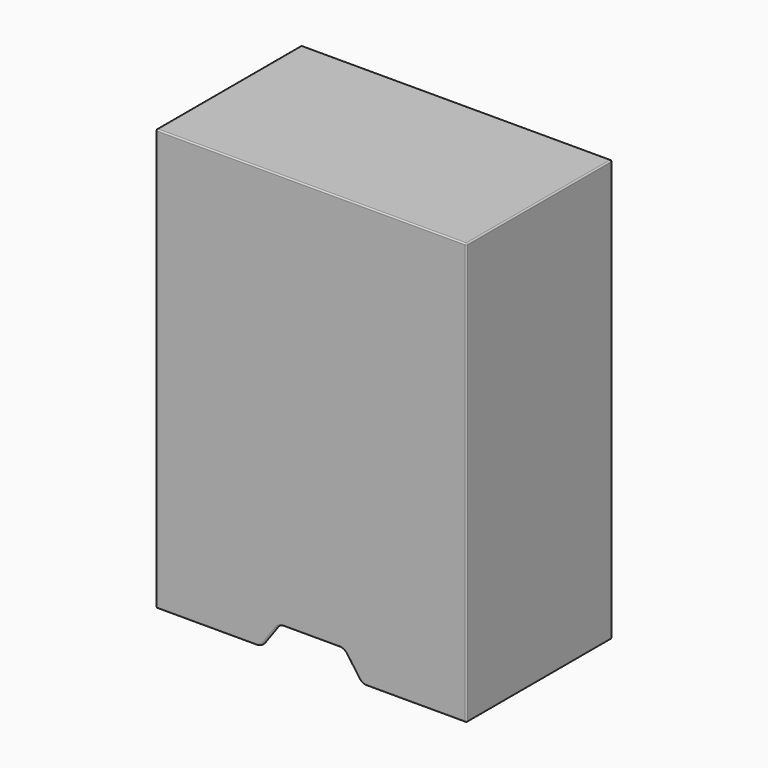
from build123d import *

# Parameters (mm, degrees)
F1_DEPTH     = 41
F2_T         = -0.5
F3_R         = 0.3
F4_T1_DEPTH  = 40.4
F4_T3_DEPTH  = 69.4
F4_T5_DEPTH  = 94.4
F4_T7_DEPTH  = 22.3555421914
F4_T9_DEPTH  = 4.9869624773
F4_T11_DEPTH = 22.2513779286
F4_T13_DEPTH = 12.4801482885
F4_T15_DEPTH = 4.9803706459
F4_S19_W     = 0.3
F4_S19_H     = 0.3
F4_T20_DEPTH = 0.3
F4_S25_W     = 0.3
F4_S25_H     = 0.3
F4_T26_DEPTH = 0.3
F4_S31_W     = 0.3
F4_S31_H     = 0.3
F4_T32_DEPTH = 0.3
F4_S37_W     = 0.3
F4_S37_H     = 0.3
F4_T38_DEPTH = 0.3
F4_S43_W     = 0.3
F4_S43_H     = 0.3
F4_T44_DEPTH = 0.3
F4_S49_W     = 0.3
F4_S49_H     = 0.3
F4_T50_DEPTH = 0.3
F4_T54_ANGLE = 54.2765520119
F4_T56_ANGLE = 54.2765520119
F4_T58_ANGLE = 54.2765520119
F4_T60_ANGLE = 54.3263722655
F4_T62_ANGLE = 54.3263722655
F4_T64_ANGLE = 54.3263722655
F4_T66_ANGLE = 54.3263722655
F4_T68_ANGLE = 54.2765520119
F4_T70_ANGLE = 90
F4_T72_ANGLE = 90


# Not quite as in the source:
# - a fillet or chamfer that OpenCascade refuses, or shapes differently, is made with other operations: its cross-section is extruded or revolved along the edge and cut away or added
# - a feature names something its author has since deleted; it is built from what else it names


with BuildPart() as f1:
    # F0 (on Front) → F1 (new body)
    with BuildSketch(Plane.XZ):
        with BuildLine():
            Line((9.8067959771, 95), (9.8067959771, 0))
            Line((9.8067959771, 0), (32.4623381684, 0))
            ThreePointArc((32.4623381684, 0), (33.3746171792, 0.2201834346), (34.086027464, 0.8322529934))
            Line((34.086027464, 0.8322529934), (36.9977827164, 4.8808917895))
            ThreePointArc((36.9977827164, 4.8808917895), (37.7091930013, 5.4929613484), (38.621472012, 5.7131447829))
            Line((38.621472012, 5.7131447829), (44.8583289981, 5.7131447829))
            Line((44.8583289981, 5.7131447829), (51.1016203005, 5.7131447829))
            ThreePointArc((51.1016203005, 5.7131447829), (52.0146730247, 5.4925645543), (52.7263243702, 4.8794795058))
            Line((52.7263243702, 4.8794795058), (55.6307139787, 0.8336652772))
            ThreePointArc((55.6307139787, 0.8336652772), (56.3423653243, 0.2205802286), (57.2554180484, 0))
            Line((57.2554180484, 0), (79.8067959771, 0))
            Line((79.8067959771, 0), (79.8067959771, 95))
            Line((79.8067959771, 95), (9.8067959771, 95))
        make_face()
    extrude(amount=F1_DEPTH)

    # F2
    f2_openings = [f1.faces().sort_by_distance(p)[0] for p in [
        (21.134567, -20.5, 0),
        (33.374617, -20.5, 0.220183),
        (35.541905, -20.5, 2.856572),
        (37.709193, -20.5, 5.492961),
        (44.861546, -20.5, 5.713145),
        (52.014673, -20.5, 5.492565),
        (56.342365, -20.5, 0.22058),
        (68.531107, -20.5, 0),
        (54.178519, -20.5, 2.856572),
    ]]
    offset(amount=F2_T, openings=f2_openings)

    # F3
    f3_edges = [f1.edges().sort_by_distance(p)[0] for p in [
        (44.806796, -41, 95),
        (9.806796, -41, 47.5),
    ]]
    fillet(f3_edges, radius=F3_R)

    # F4: fillet of radius 0.3 on 11 edges, made by hand

    # F4_s2 → F4_t1 (cut)
    with BuildSketch(Plane.XZ.offset(0.3)):
        with BuildLine():
            ThreePointArc((9.8067959771, 94.7), (9.8946639427, 94.9121320344), (10.1067959771, 95))
            Line((10.1067959771, 95), (9.8067959771, 95))
            Line((9.8067959771, 95), (9.8067959771, 94.7))
        make_face()
        with BuildLine():
            ThreePointArc((79.5067959771, 95), (79.7189280114, 94.9121320344), (79.8067959771, 94.7))
            Line((79.8067959771, 94.7), (79.8067959771, 95))
            Line((79.8067959771, 95), (79.5067959771, 95))
        make_face()
        with BuildLine():
            ThreePointArc((79.8067959771, 0.3), (79.7189280114, 0.0878679656), (79.5067959771, 0))
            Line((79.5067959771, 0), (79.8067959771, 0))
            Line((79.8067959771, 0), (79.8067959771, 0.3))
        make_face()
        with BuildLine():
            ThreePointArc((9.8067959771, 0.3), (9.8946639427, 0.0878679656), (10.1067959771, 0))
            Line((10.1067959771, 0), (9.8067959771, 0))
            Line((9.8067959771, 0), (9.8067959771, 0.3))
        make_face()
    extrude(amount=F4_T1_DEPTH, mode=Mode.SUBTRACT)

    # F4_s4 → F4_t3 (cut)
    with BuildSketch(Plane.YZ.offset(10.1067959771)):
        with BuildLine():
            ThreePointArc((-0.3, 95), (-0.0878679656, 94.9121320344), (0, 94.7))
            Line((0, 94.7), (0, 95))
            Line((0, 95), (-0.3, 95))
        make_face()
    extrude(amount=F4_T3_DEPTH, mode=Mode.SUBTRACT)

    # F4_s6 → F4_t5 (cut)
    with BuildSketch(Plane.XY.offset(0.3)):
        with BuildLine():
            ThreePointArc((9.8067959771, -0.3), (9.8946639427, -0.0878679656), (10.1067959771, 0))
            Line((10.1067959771, 0), (9.8067959771, 0))
            Line((9.8067959771, 0), (9.8067959771, -0.3))
        make_face()
        with BuildLine():
            ThreePointArc((79.5067959771, 0), (79.7189280114, -0.0878679656), (79.8067959771, -0.3))
            Line((79.8067959771, -0.3), (79.8067959771, 0))
            Line((79.8067959771, 0), (79.5067959771, 0))
        make_face()
        with BuildLine():
            ThreePointArc((79.8067959771, -40.7), (79.7189280114, -40.9121320344), (79.5067959771, -41))
            Line((79.5067959771, -41), (79.8067959771, -41))
            Line((79.8067959771, -41), (79.8067959771, -40.7))
        make_face()
    extrude(amount=F4_T5_DEPTH, mode=Mode.SUBTRACT)

    # F4_s8 → F4_t7 (cut)
    with BuildSketch(Plane.YZ.offset(10.1067959771)):
        with BuildLine():
            ThreePointArc((-40.7, 0), (-40.9121320344, 0.0878679656), (-41, 0.3))
            Line((-41, 0.3), (-41, 0))
            Line((-41, 0), (-40.7, 0))
        make_face()
        with BuildLine():
            ThreePointArc((0, 0.3), (-0.0878679656, 0.0878679656), (-0.3, 0))
            Line((-0.3, 0), (0, 0))
            Line((0, 0), (0, 0.3))
        make_face()
    extrude(amount=F4_T7_DEPTH, mode=Mode.SUBTRACT)

    # F4_s10 → F4_t9 (cut)
    with BuildSketch(Plane(origin=(12.0147086319, 0, 16.7058050126), x_dir=(0, 1, 0), z_dir=(0.5838735033, 0, 0.8118446478))):
        with BuildLine():
            ThreePointArc((-41, -26.8866284908), (-40.9121320344, -27.0987605251), (-40.7, -27.1866284908))
            Line((-40.7, -27.1866284908), (-41, -27.1866284908))
            Line((-41, -27.1866284908), (-41, -26.8866284908))
        make_face()
        with BuildLine():
            ThreePointArc((0, -26.8866284908), (-0.0878679656, -27.0987605251), (-0.3, -27.1866284908))
            Line((-0.3, -27.1866284908), (0, -27.1866284908))
            Line((0, -27.1866284908), (0, -26.8866284908))
        make_face()
    extrude(amount=F4_T9_DEPTH, mode=Mode.SUBTRACT)

    # F4_s12 → F4_t11 (cut)
    with BuildSketch(Plane.YZ.offset(57.2554180484)):
        with BuildLine():
            ThreePointArc((-41, 0.3), (-40.9121320344, 0.0878679656), (-40.7, 0))
            Line((-40.7, 0), (-41, 0))
            Line((-41, 0), (-41, 0.3))
        make_face()
        with BuildLine():
            ThreePointArc((0, 0.3), (-0.0878679656, 0.0878679656), (-0.3, 0))
            Line((-0.3, 0), (0, 0))
            Line((0, 0), (0, 0.3))
        make_face()
    extrude(amount=F4_T11_DEPTH, mode=Mode.SUBTRACT)

    # F4_s14 → F4_t13 (cut)
    with BuildSketch(Plane.YZ.offset(38.621472012)):
        with BuildLine():
            ThreePointArc((0, 6.0131447829), (-0.0878679656, 5.8010127486), (-0.3, 5.7131447829))
            Line((-0.3, 5.7131447829), (0, 5.7131447829))
            Line((0, 5.7131447829), (0, 6.0131447829))
        make_face()
        with BuildLine():
            ThreePointArc((-41, 6.0131447829), (-40.9121320344, 5.8010127486), (-40.7, 5.7131447829))
            Line((-40.7, 5.7131447829), (-41, 5.7131447829))
            Line((-41, 5.7131447829), (-41, 6.0131447829))
        make_face()
    extrude(amount=F4_T13_DEPTH, mode=Mode.SUBTRACT)

    # F4_s16 → F4_t15 (cut)
    with BuildSketch(Plane(origin=(15.6197974129, 0, -21.7583751289), x_dir=(0, 1, 0), z_dir=(0.5831673614, 0, -0.8123520349))):
        with BuildLine():
            ThreePointArc((0, 45.9778900823), (-0.0878679656, 45.765758048), (-0.3, 45.6778900823))
            Line((-0.3, 45.6778900823), (0, 45.6778900823))
            Line((0, 45.6778900823), (0, 45.9778900823))
        make_face()
        with BuildLine():
            ThreePointArc((-41, 45.9778900823), (-40.9121320344, 45.765758048), (-40.7, 45.6778900823))
            Line((-40.7, 45.6778900823), (-41, 45.6778900823))
            Line((-41, 45.6778900823), (-41, 45.9778900823))
        make_face()
    extrude(amount=F4_T15_DEPTH, mode=Mode.SUBTRACT)


with BuildPart() as f4_tool18:
    # F4_s19 → F4_t20 (new body)
    with BuildSketch(Plane.YZ.offset(10.1067959771)):
        with Locations((-40.85, 94.85)):
            Rectangle(F4_S19_W, F4_S19_H)
    extrude(amount=-F4_T20_DEPTH)

    # F4_s21 → F4_t22 (revolve, cut)
    with BuildSketch(Plane(origin=(10.1067959771, -40.7, 94.7), x_dir=(0, 0.7071067812, -0.7071067812), z_dir=(0, 0.7071067812, 0.7071067812))):
        with BuildLine():
            ThreePointArc((0, -0.3), (0.3, 0), (0, 0.3))
            Line((0, 0.3), (0, -0.3))
        make_face()
    revolve(axis=Axis((10.1067959771, -40.7, 94.7), (-1, 0, 0)), mode=Mode.SUBTRACT)


with BuildPart() as f1_1:
    add(f1.part)

    # F4_t17: cut F4_tool18
    add(f4_tool18.part, mode=Mode.SUBTRACT)


with BuildPart() as f4_tool24:
    # F4_s25 → F4_t26 (new body)
    with BuildSketch(Plane.YZ.offset(10.1067959771)):
        with Locations((-0.15, 94.85)):
            Rectangle(F4_S25_W, F4_S25_H)
    extrude(amount=-F4_T26_DEPTH)

    # F4_s27 → F4_t28 (revolve, cut)
    with BuildSketch(Plane(origin=(10.1067959771, -0.3, 94.7), x_dir=(0, -0.7071067812, -0.7071067812), z_dir=(0, 0.7071067812, -0.7071067812))):
        with BuildLine():
            ThreePointArc((0, -0.3), (0.3, 0), (0, 0.3))
            Line((0, 0.3), (0, -0.3))
        make_face()
    revolve(axis=Axis((10.1067959771, -0.3, 94.7), (-1, 0, 0)), mode=Mode.SUBTRACT)


with BuildPart() as f1_2:
    add(f1_1.part)

    # F4_t23: cut F4_tool24
    add(f4_tool24.part, mode=Mode.SUBTRACT)


with BuildPart() as f4_tool30:
    # F4_s31 → F4_t32 (new body)
    with BuildSketch(Plane.XY.offset(94.7)):
        with Locations((79.6567959771, -0.15)):
            Rectangle(F4_S31_W, F4_S31_H)
    extrude(amount=F4_T32_DEPTH)

    # F4_s33 → F4_t34 (revolve, cut)
    with BuildSketch(Plane(origin=(79.5067959771, -0.3, 94.7), x_dir=(-0.7071067812, -0.7071067812, 0), z_dir=(-0.7071067812, 0.7071067812, 0))):
        with BuildLine():
            ThreePointArc((0, -0.3), (0.3, 0), (0, 0.3))
            Line((0, 0.3), (0, -0.3))
        make_face()
    revolve(axis=Axis((79.5067959771, -0.3, 94.7), (0, 0, 1)), mode=Mode.SUBTRACT)


with BuildPart() as f1_3:
    add(f1_2.part)

    # F4_t29: cut F4_tool30
    add(f4_tool30.part, mode=Mode.SUBTRACT)


with BuildPart() as f4_tool36:
    # F4_s37 → F4_t38 (new body)
    with BuildSketch(Plane.YZ.offset(10.1067959771)):
        with Locations((-0.15, 0.15)):
            Rectangle(F4_S37_W, F4_S37_H)
    extrude(amount=-F4_T38_DEPTH)

    # F4_s39 → F4_t40 (revolve, cut)
    with BuildSketch(Plane(origin=(10.1067959771, -0.3, 0.3), x_dir=(0, -0.7071067812, 0.7071067812), z_dir=(0, -0.7071067812, -0.7071067812))):
        with BuildLine():
            ThreePointArc((0, -0.3), (0.3, 0), (0, 0.3))
            Line((0, 0.3), (0, -0.3))
        make_face()
    revolve(axis=Axis((10.1067959771, -0.3, 0.3), (-1, 0, 0)), mode=Mode.SUBTRACT)


with BuildPart() as f1_4:
    add(f1_3.part)

    # F4_t35: cut F4_tool36
    add(f4_tool36.part, mode=Mode.SUBTRACT)


with BuildPart() as f4_tool42:
    # F4_s43 → F4_t44 (new body)
    with BuildSketch(Plane.XZ.offset(0.3)):
        with Locations((79.6567959771, 0.15)):
            Rectangle(F4_S43_W, F4_S43_H)
    extrude(amount=-F4_T44_DEPTH)

    # F4_s45 → F4_t46 (revolve, cut)
    with BuildSketch(Plane(origin=(79.5067959771, -0.3, 0.3), x_dir=(-0.7071067812, 0, 0.7071067812), z_dir=(-0.7071067812, 0, -0.7071067812))):
        with BuildLine():
            ThreePointArc((0, -0.3), (0.3, 0), (0, 0.3))
            Line((0, 0.3), (0, -0.3))
        make_face()
    revolve(axis=Axis((79.5067959771, -0.3, 0.3), (0, 1, 0)), mode=Mode.SUBTRACT)


with BuildPart() as f1_5:
    add(f1_4.part)

    # F4_t41: cut F4_tool42
    add(f4_tool42.part, mode=Mode.SUBTRACT)


with BuildPart() as f4_tool48:
    # F4_s49 → F4_t50 (new body)
    with BuildSketch(Plane.XY.offset(0.3)):
        with Locations((79.6567959771, -40.85)):
            Rectangle(F4_S49_W, F4_S49_H)
    extrude(amount=-F4_T50_DEPTH)

    # F4_s51 → F4_t52 (revolve, cut)
    with BuildSketch(Plane(origin=(79.5067959771, -40.7, 0.3), x_dir=(-0.7071067812, 0.7071067812, 0), z_dir=(-0.7071067812, -0.7071067812, 0))):
        with BuildLine():
            ThreePointArc((0, -0.3), (0.3, 0), (0, 0.3))
            Line((0, 0.3), (0, -0.3))
        make_face()
    revolve(axis=Axis((79.5067959771, -40.7, 0.3), (0, 0, -1)), mode=Mode.SUBTRACT)


with BuildPart() as f1_6:
    add(f1_5.part)

    # F4_t47: cut F4_tool48
    add(f4_tool48.part, mode=Mode.SUBTRACT)

    # F4_s53 → F4_t54 (revolve, cut)
    with BuildSketch(Plane.YZ.offset(32.4623381684)):
        with BuildLine():
            ThreePointArc((-41, 0.3), (-40.9121320344, 0.0878679656), (-40.7, 0))
            Line((-40.7, 0), (-41, 0))
            Line((-41, 0), (-41, 0.3))
        make_face()
    revolve(axis=Axis((32.4623381684, -41, 2), (0, -1, 0)), revolution_arc=F4_T54_ANGLE, mode=Mode.SUBTRACT)

    # F4_s55 → F4_t56 (revolve, cut)
    with BuildSketch(Plane.YZ.offset(32.4623381684)):
        with BuildLine():
            ThreePointArc((0, 0.3), (-0.0878679656, 0.0878679656), (-0.3, 0))
            Line((-0.3, 0), (0, 0))
            Line((0, 0), (0, 0.3))
        make_face()
    revolve(axis=Axis((32.4623381684, 0, 2), (0, -1, 0)), revolution_arc=F4_T56_ANGLE, mode=Mode.SUBTRACT)

    # F4_s57 → F4_t58 (revolve, cut)
    with BuildSketch(Plane(origin=(14.9264638842, 0, 20.7544438086), x_dir=(0, 1, 0), z_dir=(-0.5838735033, 0, -0.8118446478))):
        with BuildLine():
            ThreePointArc((0, 26.8866284908), (-0.0878679656, 27.0987605251), (-0.3, 27.1866284908))
            Line((-0.3, 27.1866284908), (0, 27.1866284908))
            Line((0, 27.1866284908), (0, 26.8866284908))
        make_face()
    revolve(axis=Axis((38.621472012, 0, 3.7131447829), (0, 1, 0)), revolution_arc=F4_T58_ANGLE, mode=Mode.SUBTRACT)

    # F4_s59 → F4_t60 (revolve, cut)
    with BuildSketch(Plane.YZ.offset(51.1016203005)):
        with BuildLine():
            ThreePointArc((0, 6.0131447829), (-0.0878679656, 5.8010127486), (-0.3, 5.7131447829))
            Line((-0.3, 5.7131447829), (0, 5.7131447829))
            Line((0, 5.7131447829), (0, 6.0131447829))
        make_face()
    revolve(axis=Axis((51.1016203005, 0, 3.7131447829), (0, 1, 0)), revolution_arc=F4_T60_ANGLE, mode=Mode.SUBTRACT)

    # F4_s61 → F4_t62 (revolve, cut)
    with BuildSketch(Plane(origin=(18.5241870214, 0, -25.8041893575), x_dir=(0, 1, 0), z_dir=(-0.5831673614, 0, 0.8123520349))):
        with BuildLine():
            ThreePointArc((0, -45.9778900823), (-0.0878679656, -45.765758048), (-0.3, -45.6778900823))
            Line((-0.3, -45.6778900823), (0, -45.6778900823))
            Line((0, -45.6778900823), (0, -45.9778900823))
        make_face()
    revolve(axis=Axis((57.2554180484, 0, 2), (0, -1, 0)), revolution_arc=F4_T62_ANGLE, mode=Mode.SUBTRACT)

    # F4_s63 → F4_t64 (revolve, cut)
    with BuildSketch(Plane(origin=(18.5241870214, 0, -25.8041893575), x_dir=(0, 1, 0), z_dir=(-0.5831673614, 0, 0.8123520349))):
        with BuildLine():
            ThreePointArc((-41, -45.9778900823), (-40.9121320344, -45.765758048), (-40.7, -45.6778900823))
            Line((-40.7, -45.6778900823), (-41, -45.6778900823))
            Line((-41, -45.6778900823), (-41, -45.9778900823))
        make_face()
    revolve(axis=Axis((57.2554180484, -41, 2), (0, -1, 0)), revolution_arc=F4_T64_ANGLE, mode=Mode.SUBTRACT)

    # F4_s65 → F4_t66 (revolve, cut)
    with BuildSketch(Plane.YZ.offset(51.1016203005)):
        with BuildLine():
            ThreePointArc((-41, 6.0131447829), (-40.9121320344, 5.8010127486), (-40.7, 5.7131447829))
            Line((-40.7, 5.7131447829), (-41, 5.7131447829))
            Line((-41, 5.7131447829), (-41, 6.0131447829))
        make_face()
    revolve(axis=Axis((51.1016203005, -41, 3.7131447829), (0, 1, 0)), revolution_arc=F4_T66_ANGLE, mode=Mode.SUBTRACT)

    # F4_s67 → F4_t68 (revolve, cut)
    with BuildSketch(Plane(origin=(14.9264638842, 0, 20.7544438086), x_dir=(0, 1, 0), z_dir=(-0.5838735033, 0, -0.8118446478))):
        with BuildLine():
            ThreePointArc((-41, 26.8866284908), (-40.9121320344, 27.0987605251), (-40.7, 27.1866284908))
            Line((-40.7, 27.1866284908), (-41, 27.1866284908))
            Line((-41, 27.1866284908), (-41, 26.8866284908))
        make_face()
    revolve(axis=Axis((38.621472012, -41, 3.7131447829), (0, 1, 0)), revolution_arc=F4_T68_ANGLE, mode=Mode.SUBTRACT)

    # F4_s69 → F4_t70 (revolve, cut)
    with BuildSketch(Plane.XZ.offset(40.7)):
        with BuildLine():
            ThreePointArc((9.8067959771, 0.3), (9.8946639427, 0.0878679656), (10.1067959771, 0))
            Line((10.1067959771, 0), (9.8067959771, 0))
            Line((9.8067959771, 0), (9.8067959771, 0.3))
        make_face()
    revolve(axis=Axis((10.1067959771, -40.7, 0), (0, 0, 1)), revolution_arc=F4_T70_ANGLE, mode=Mode.SUBTRACT)

    # F4_s71 → F4_t72 (revolve, cut)
    with BuildSketch(Plane.XY.offset(94.7)):
        with BuildLine():
            ThreePointArc((79.8067959771, -40.7), (79.7189280114, -40.9121320344), (79.5067959771, -41))
            Line((79.5067959771, -41), (79.8067959771, -41))
            Line((79.8067959771, -41), (79.8067959771, -40.7))
        make_face()
    revolve(axis=Axis((79.8067959771, -40.7, 94.7), (-1, 0, 0)), revolution_arc=F4_T72_ANGLE, mode=Mode.SUBTRACT)


solid = f1_6.part
